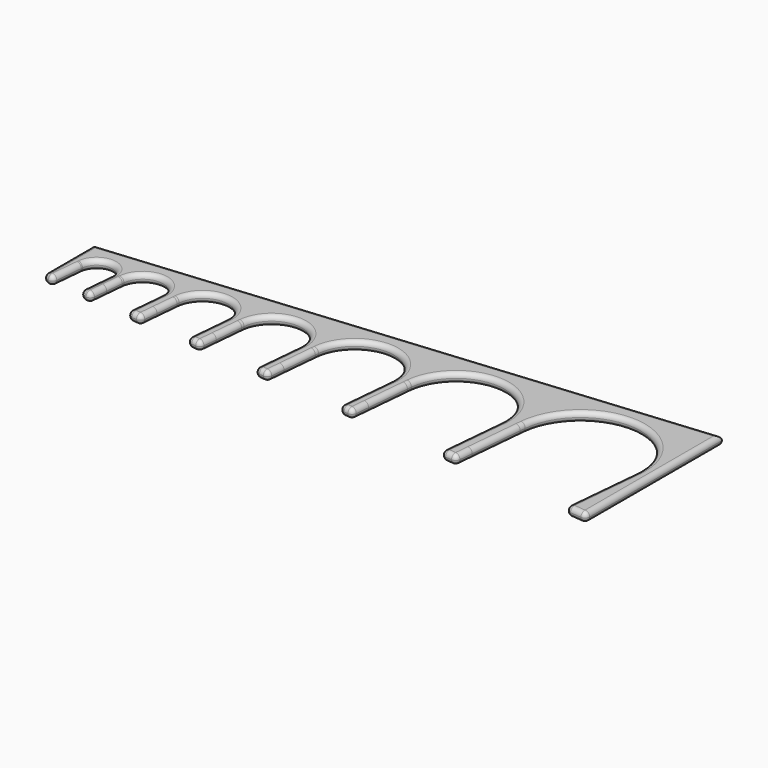
from build123d import *

# Parameters (mm, degrees)
F1_DEPTH = 2
F2_R     = 0.99999


# Not quite as in the source:
# - a fillet or chamfer is up to 0.001 mm smaller than in the source, because OpenCascade refuses the exact size


with BuildPart() as f1:
    # F0 (on Top) → F1 (new body)
    with BuildSketch(Plane.XY):
        with BuildLine():
            ThreePointArc((-4.3813439977, 0.4047527312), (0.2025912263, 4.3953335249), (4.4, 0))
            Line((4.4, 0), (7.4765806993, 0))
            Line((7.4765806993, 0), (7.5233200028, 0.505940914))
            ThreePointArc((7.5233200028, 0.505940914), (13.2532390328, 5.4941669061), (18.5, 0))
            Line((18.5, 0), (21.4723226447, 0))
            Line((21.4723226447, 0), (21.5275600033, 0.5979301711))
            ThreePointArc((21.5275600033, 0.5979301711), (28.2992824934, 6.4931063436), (34.5, 0))
            Line((34.5, 0), (37.4638065353, 0))
            Line((37.4638065353, 0), (37.5360400044, 0.7819086853))
            ThreePointArc((37.5360400044, 0.7819086853), (46.3913694144, 8.4909852185), (54.5, 0))
            Line((54.5, 0), (57.455290426, 0))
            Line((57.455290426, 0), (57.5445200054, 0.9658871995))
            ThreePointArc((57.5445200054, 0.9658871995), (68.4834563354, 10.4888640935), (78.5, 0))
            Line((78.5, 0), (81.9446452893, 0))
            Line((81.9446452893, 0), (82.0551200067, 1.1958603422))
            ThreePointArc((82.0551200067, 1.1958603422), (95.5985649867, 12.9862126872), (108, 0))
            Line((108, 0), (110.9048114853, 0))
            Line((110.9048114853, 0), (110.9048114853, 18.4863338511))
            Line((110.9048114853, 18.4863338511), (-16, 6.7627465044))
            Line((-16, 6.7627465044), (-16, 0))
            Line((-16, 0), (-13.3140515804, 0))
            Line((-13.3140515804, 0), (-13.2860079983, 0.3035645484))
            ThreePointArc((-13.2860079983, 0.3035645484), (-9.8480565803, 3.2965001437), (-6.7, 0))
            Line((-6.7, 0), (-4.4187354405, 0))
            Line((-4.4187354405, 0), (-4.3813439977, 0.4047527312))
        make_face()
        Polygon((-13.9562424613, -6.9515507722), (-13.3140515804, 0), (-16, 0), (-16, -6.7627465044), align=None)
        with BuildLine():
            Line((-4.7682416665, -3.7833148175), (-4.4187354405, 0))
            Line((-4.4187354405, 0), (-6.7, 0))
            ThreePointArc((-6.7, 0), (-6.7034998563, -0.1519434197), (-6.7139920017, -0.3035645484))
            Line((-6.7139920017, -0.3035645484), (-7.0162694363, -3.5756398711))
            Line((-7.0162694363, -3.5756398711), (-4.7682416665, -3.7833148175))
        make_face()
        Polygon((-5.1361986949, -7.7663548154), (-4.7682416665, -3.7833148175), (-7.0162694363, -3.5756398711), (-7.3842264646, -7.5586798691), align=None)
        with BuildLine():
            Line((7.4765806993, 0), (4.4, 0))
            ThreePointArc((4.4, 0), (4.3953335249, -0.2025912263), (4.3813439977, -0.4047527312))
            Line((4.3813439977, -0.4047527312), (3.994446329, -4.5928202799))
            Line((3.994446329, -4.5928202799), (7.0264160296, -4.8729165284))
            Line((7.0264160296, -4.8729165284), (7.4765806993, 0))
        make_face()
        Polygon((7.0264160296, -4.8729165284), (3.994446329, -4.5928202799), (3.6264893006, -8.5758602779), (6.6584590012, -8.8559565264), align=None)
        with BuildLine():
            Line((21.4723226447, 0), (18.5, 0))
            ThreePointArc((18.5, 0), (18.4941669061, -0.2532390328), (18.4766799972, -0.505940914))
            Line((18.4766799972, -0.505940914), (17.9797760239, -5.8847983565))
            Line((17.9797760239, -5.8847983565), (20.9037256788, -6.1549156103))
            Line((20.9037256788, -6.1549156103), (21.4723226447, 0))
        make_face()
        Polygon((20.9037256788, -6.1549156103), (17.9797760239, -5.8847983565), (17.6118189955, -9.8678383544), (20.5357686504, -10.1379556083), align=None)
        with BuildLine():
            Line((37.4638065353, 0), (34.5, 0))
            ThreePointArc((34.5, 0), (34.4931063436, -0.2992824934), (34.4724399967, -0.5979301711))
            Line((34.4724399967, -0.5979301711), (33.8486056721, -7.3507759526))
            Line((33.8486056721, -7.3507759526), (36.7598892582, -7.6197231029))
            Line((36.7598892582, -7.6197231029), (37.4638065353, 0))
        make_face()
        Polygon((36.7598892582, -7.6197231029), (33.8486056721, -7.3507759526), (33.4806486437, -11.3338159505), (36.3919322298, -11.6027631009), align=None)
        with BuildLine():
            Line((57.455290426, 0), (54.5, 0))
            ThreePointArc((54.5, 0), (54.4909852185, -0.3913694144), (54.4639599956, -0.7819086853))
            Line((54.4639599956, -0.7819086853), (53.6878092495, -9.1835404735))
            Line((53.6878092495, -9.1835404735), (56.582204744, -9.4509274859))
            Line((56.582204744, -9.4509274859), (57.455290426, 0))
        make_face()
        Polygon((56.582204744, -9.4509274859), (53.6878092495, -9.1835404735), (53.3198522211, -13.1665804715), (56.2142477156, -13.4339674838), align=None)
        with BuildLine():
            Line((81.9446452893, 0), (78.5, 0))
            ThreePointArc((78.5, 0), (78.4888640935, -0.4834563354), (78.4554799946, -0.9658871995))
            Line((78.4554799946, -0.9658871995), (77.4931647332, -11.3827018849))
            Line((77.4931647332, -11.3827018849), (80.8643301129, -11.6941333533))
            Line((80.8643301129, -11.6941333533), (81.9446452893, 0))
        make_face()
        Polygon((77.1252077048, -15.3657418828), (80.4963730845, -15.6771733512), (80.8643301129, -11.6941333533), (77.4931647332, -11.3827018849), align=None)
        with BuildLine():
            Line((110.9048114853, -18.4863338511), (110.9048114853, 0))
            Line((110.9048114853, 0), (108, 0))
            ThreePointArc((108, 0), (107.9862126872, -0.5985649867), (107.9448799933, -1.1958603422))
            Line((107.9448799933, -1.1958603422), (106.3861330712, -18.0688940357))
            Line((106.3861330712, -18.0688940357), (110.9048114853, -18.4863338511))
        make_face()
    extrude(amount=F1_DEPTH)

    # F2 (radius 1 in the source; OpenCascade refuses exactly that, so slightly less here)
    f2_edges = [f1.edges().sort_by_distance(p)[0] for p in [
        (47.452406, 12.62454, 2),
        (-16, 0, 2),
        (-14.978121, -6.857149, 2),
        (-13.621125, -3.323993, 2),
        (-9.696435, 3.286008, 2),
        (-7.049109, -3.931122, 2),
        (-6.260213, -7.662517, 2),
        (-4.758771, -3.680801, 2),
        (0.404753, 4.381344, 2),
        (4.003917, -4.490307, 2),
        (5.142474, -8.715908, 2),
        (7.09089, -4.175008, 2),
        (13.505941, 5.47668, 2),
        (18.044249, -5.18689, 2),
        (19.073794, -10.002897, 2),
        (21.031664, -4.770013, 2),
        (28.59793, 6.47244, 2),
        (33.976544, -5.965873, 2),
        (34.93629, -11.46829, 2),
        (36.963986, -5.410427, 2),
        (46.781909, 8.46396, 2),
        (53.891906, -6.974245, 2),
        (54.76705, -13.300274, 2),
        (56.879384, -6.23404, 2),
        (68.965887, 10.45548, 2),
        (77.790344, -8.165815, 2),
        (78.81079, -15.521458, 2),
        (81.275747, -7.240657, 2),
        (96.19586, 12.94488, 2),
        (107.165507, -9.632377, 2),
        (108.645472, -18.277614, 2),
        (110.904811, 0, 2),
        (47.452406, 12.62454, 0),
        (-16, 0, 0),
        (-14.978121, -6.857149, 0),
        (-13.621125, -3.323993, 0),
        (-9.696435, 3.286008, 0),
        (-7.049109, -3.931122, 0),
        (-6.260213, -7.662517, 0),
        (-4.758771, -3.680801, 0),
        (0.404753, 4.381344, 0),
        (4.003917, -4.490307, 0),
        (5.142474, -8.715908, 0),
        (7.09089, -4.175008, 0),
        (13.505941, 5.47668, 0),
        (18.044249, -5.18689, 0),
        (19.073794, -10.002897, 0),
        (21.031664, -4.770013, 0),
        (28.59793, 6.47244, 0),
        (33.976544, -5.965873, 0),
        (34.93629, -11.46829, 0),
        (36.963986, -5.410427, 0),
        (46.781909, 8.46396, 0),
        (53.891906, -6.974245, 0),
        (54.76705, -13.300274, 0),
        (56.879384, -6.23404, 0),
        (68.965887, 10.45548, 0),
        (77.790344, -8.165815, 0),
        (78.81079, -15.521458, 0),
        (81.275747, -7.240657, 0),
        (96.19586, 12.94488, 0),
        (107.165507, -9.632377, 0),
        (108.645472, -18.277614, 0),
        (110.904811, 0, 0),
        (-13.956242, -6.951551, 1),
        (-16, -6.762747, 1),
        (-7.384226, -7.55868, 1),
        (-5.136199, -7.766355, 1),
        (3.626489, -8.57586, 1),
        (6.658459, -8.855957, 1),
        (20.535769, -10.137956, 1),
        (17.611819, -9.867838, 1),
        (33.480649, -11.333816, 1),
        (36.391932, -11.602763, 1),
        (53.319852, -13.16658, 1),
        (56.214248, -13.433967, 1),
        (80.496373, -15.677173, 1),
        (77.125208, -15.365742, 1),
        (110.904811, -18.486334, 1),
        (106.386133, -18.068894, 1),
    ]]
    fillet(f2_edges, radius=F2_R)


solid = f1.part
